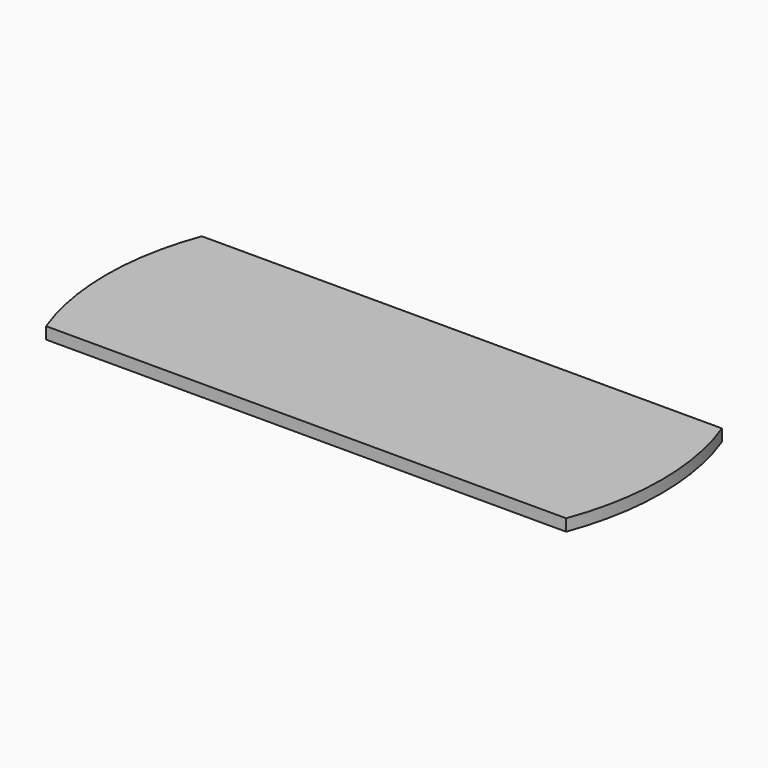
from build123d import *

# Parameters (mm, degrees)
F1_DEPTH = 0.2
F2_DEPTH = 1.2


# Not quite as in the source:
# - a feature names something its author has since deleted; it is built from what else it names


with BuildPart() as f1:
    # F0 (on Top) → F1 (new body)
    with BuildSketch(Plane.XY):
        with BuildLine():
            Line((0, -15), (-30.3973683071, -15))
            ThreePointArc((-30.3973683071, -15), (-32.5, -26.5), (-30.3973683071, -38))
            Line((-30.3973683071, -38), (0, -38))
            Line((0, -38), (30.3973683071, -38))
            ThreePointArc((30.3973683071, -38), (32.5, -26.5), (30.3973683071, -15))
            Line((30.3973683071, -15), (0, -15))
        make_face()
        with BuildLine():
            Line((30.7179100852, -15), (30.3973683071, -15))
            ThreePointArc((30.3973683071, -15), (32.5, -26.5), (30.3973683071, -38))
            Line((30.3973683071, -38), (30.7179100852, -38))
            ThreePointArc((30.7179100852, -38), (32.8, -26.5), (30.7179100852, -15))
        make_face()
        with BuildLine():
            ThreePointArc((-30.3973683071, -38), (-32.5, -26.5), (-30.3973683071, -15))
            Line((-30.3973683071, -15), (-30.7179100852, -15))
            ThreePointArc((-30.7179100852, -15), (-32.8, -26.5), (-30.7179100852, -38))
            Line((-30.7179100852, -38), (-30.3973683071, -38))
        make_face()
    extrude(amount=-F1_DEPTH)

    # F0 (on Top) → F2 (join)
    with BuildSketch(Plane.XY):
        with BuildLine():
            ThreePointArc((-30.3973683071, -38), (-32.5, -26.5), (-30.3973683071, -15))
            Line((-30.3973683071, -15), (-30.7179100852, -15))
            ThreePointArc((-30.7179100852, -15), (-32.8, -26.5), (-30.7179100852, -38))
            Line((-30.7179100852, -38), (-30.3973683071, -38))
        make_face()
        with BuildLine():
            Line((30.7179100852, -15), (30.3973683071, -15))
            ThreePointArc((30.3973683071, -15), (32.5, -26.5), (30.3973683071, -38))
            Line((30.3973683071, -38), (30.7179100852, -38))
            ThreePointArc((30.7179100852, -38), (32.8, -26.5), (30.7179100852, -15))
        make_face()
        with BuildLine():
            Line((0, -15), (-30.3973683071, -15))
            ThreePointArc((-30.3973683071, -15), (-32.5, -26.5), (-30.3973683071, -38))
            Line((-30.3973683071, -38), (0, -38))
            Line((0, -38), (30.3973683071, -38))
            ThreePointArc((30.3973683071, -38), (32.5, -26.5), (30.3973683071, -15))
            Line((30.3973683071, -15), (0, -15))
        make_face()
    extrude(amount=F2_DEPTH)


solid = f1.part
